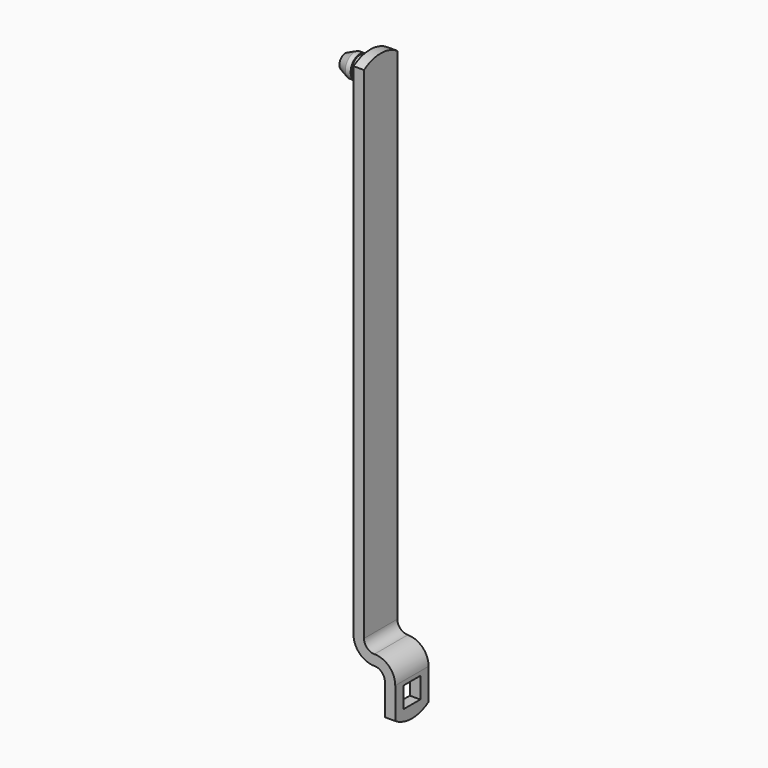
from build123d import *

# Parameters (mm, degrees)
F0_W      = 5
F0_H      = 15
F1_DEPTH  = 20
F3_DEPTH  = 5
F2_W      = 10
F2_H      = 10
F4_DEPTH  = 20.001
F6_DEPTH  = 5
F5_R      = 5
F7_DEPTH  = 5
F8_R      = 5.5
F8_R_2    = 5
F9_DEPTH  = 2.5
F11_R     = 3.5
F9_FACE_R = 5.5


with BuildPart() as f1:
    # F0 (on Front) → F1 (new body)
    with BuildSketch(Plane.XZ):
        with BuildLine():
            ThreePointArc((7.5, -125), (3.9644660941, -123.5355339059), (2.5, -120))
            Line((2.5, -120), (-2.5, -120))
            ThreePointArc((-2.5, -120), (-1.6143782777, -124.1143782777), (0.8856217223, -127.5))
            ThreePointArc((0.8856217223, -127.5), (3.9644660941, -125.6458565331), (7.5, -125))
        make_face()
        with BuildLine():
            Line((-2.5, -120), (2.5, -120))
            Line((2.5, -120), (2.5, -111.3397459622))
            ThreePointArc((2.5, -111.3397459622), (-1.1602540378, -115), (-2.5, -120))
        make_face()
        with BuildLine():
            Line((-2.5, 120), (-2.5, -120))
            ThreePointArc((-2.5, -120), (-1.1602540378, -115), (2.5, -111.3397459622))
            Line((2.5, -111.3397459622), (2.5, 120))
            Line((2.5, 120), (-2.5, 120))
        make_face()
        with BuildLine():
            ThreePointArc((17.5, -135), (14.5710678119, -127.9289321881), (7.5, -125))
            Line((7.5, -125), (7.5, -130))
            ThreePointArc((7.5, -130), (11.0355339059, -131.4644660941), (12.5, -135))
            Line((12.5, -135), (17.5, -135))
        make_face()
        with BuildLine():
            Line((7.5, -130), (7.5, -125))
            ThreePointArc((7.5, -125), (3.9644660941, -125.6458565331), (0.8856217223, -127.5))
            ThreePointArc((0.8856217223, -127.5), (3.9644660941, -129.3541434669), (7.5, -130))
        make_face()
        with Locations((15, -142.5)):
            Rectangle(F0_W, F0_H)
    extrude(amount=F1_DEPTH)

    # F2 (on face) → F3 (join)
    with BuildSketch(Plane.YZ.offset(17.5)):
        with BuildLine():
            Line((0, -150), (-20, -150))
            ThreePointArc((-20, -150), (-10, -153), (0, -150))
        make_face()
    extrude(amount=-F3_DEPTH)

    # F2 (on face) → F4 (cut, through all)
    with BuildSketch(Plane.YZ.offset(17.5)):
        with Locations((-10, -142)):
            Rectangle(F2_W, F2_H)
    extrude(amount=-F4_DEPTH, mode=Mode.SUBTRACT)

    # F5 (on face) → F6 (join)
    with BuildSketch(Plane(origin=(-2.5, 0, 0), x_dir=(0, -1, 0), z_dir=(-1, 0, 0))):
        with BuildLine():
            Line((0, 120), (20, 120))
            ThreePointArc((20, 120), (10, 123), (0, 120))
        make_face()
    extrude(amount=-F6_DEPTH)

    # F5 (on face) → F7 (join)
    with BuildSketch(Plane(origin=(-2.5, 0, 0), x_dir=(0, -1, 0), z_dir=(-1, 0, 0))):
        with Locations((10, 114)):
            Circle(F5_R)
    extrude(amount=F7_DEPTH)

    # F8 (on face) → F9 (join)
    with BuildSketch(Plane(origin=(-7.5, 0, 0), x_dir=(0, -1, 0), z_dir=(-1, 0, 0))):
        with Locations((10, 114)):
            Circle(F8_R)
        with Locations((10, 114)):
            Circle(F8_R_2, mode=Mode.SUBTRACT)
        with Locations((10, 114)):
            Circle(F8_R_2)
    extrude(amount=F9_DEPTH)

    # F11 (on offset) → F12 section 0
    with BuildSketch(Plane(origin=(-14.5, 0, 0), x_dir=(0, -1, 0), z_dir=(-1, 0, 0))):
        with Locations((10, 114)):
            Circle(F11_R)
    # F9_face (on face) → F12 section 1
    with BuildSketch(Plane(origin=(-10, -10, 114), x_dir=(0, -1, 0), z_dir=(-1, 0, 0))):
        Circle(F9_FACE_R)
    loft()


solid = f1.part
